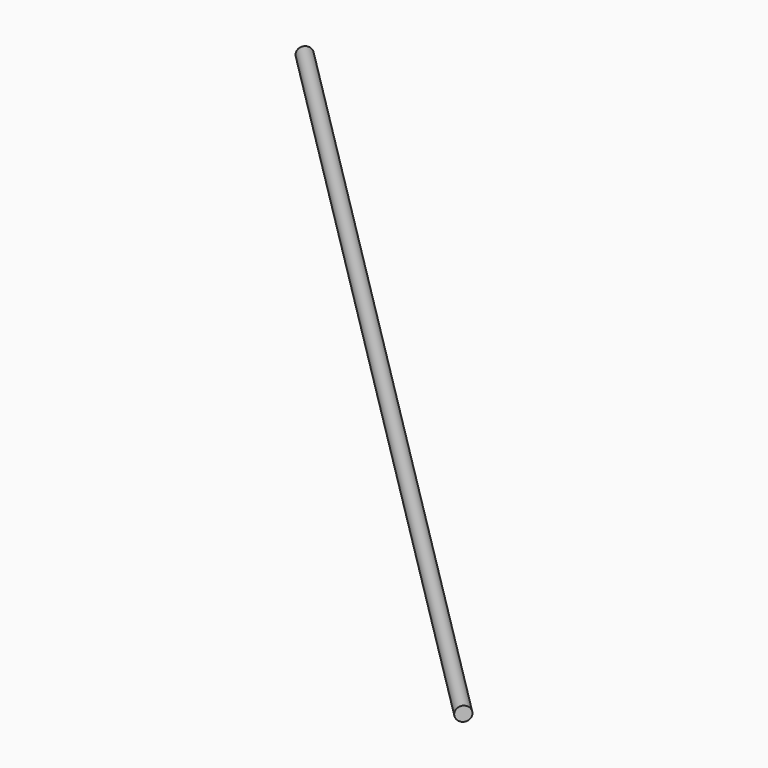
from build123d import *

# Parameters (mm, degrees)
F0_R     = 9.525
F1_DEPTH = 1489.075
F3_ANGLE = 45


# Not quite as in the source:
# - a feature names something its author has since deleted; it is built from what else it names


with BuildPart() as f1:
    # F0 (on Front) → F1 (new body)
    with BuildSketch(Plane.XZ):
        Circle(F0_R)
    extrude(amount=F1_DEPTH)


with BuildPart() as f1_1:
    # F3: moved
    add(f1.part.rotate(Axis((0, 0, 6.35), (0, 0, 1)), F3_ANGLE))


solid = f1_1.part
